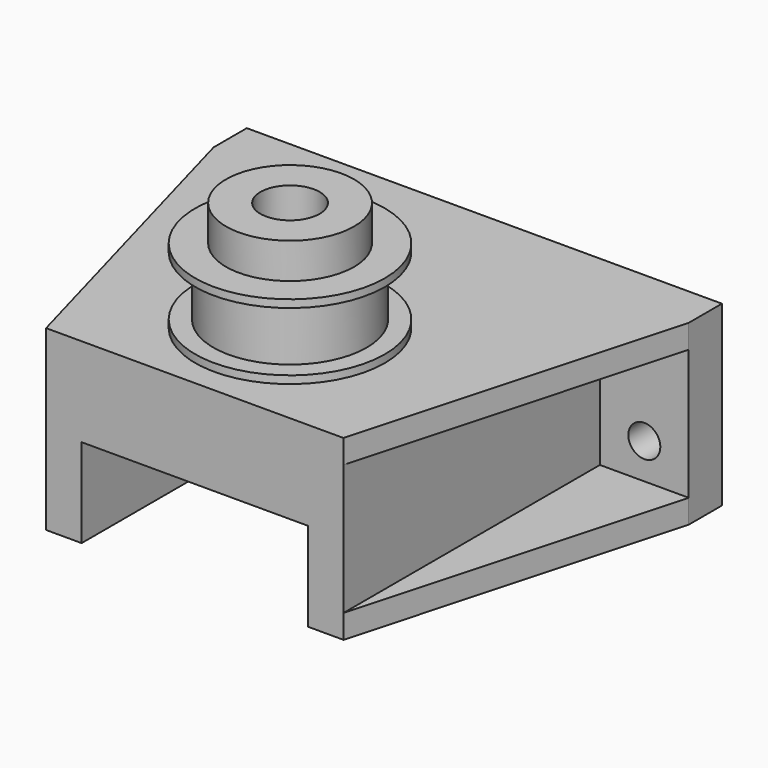
from build123d import *

# Parameters (mm, degrees)
F0_W              = 50.2
F0_H              = 61.1
F0_R              = 15.1
F1_DEPTH          = 15
F2_R              = 15
F2_R_2            = 5
F3_DEPTH          = 14
F5_DEPTH          = 15
F6_W              = 7
F6_H              = 30
F7_DEPTH          = 15
F8_R              = 2.7
F9_DEPTH          = 25
F11_DEPTH         = 4
F11_COPIES2_COUNT = 2
F12_R             = 16
F12_R_2           = 5
F13_DEPTH         = 1.3
F14_R             = 12.9361137745
F14_R_2           = 5
F15_DEPTH         = 10
F16_R             = 16
F16_R_2           = 5
F17_DEPTH         = 1.3
F18_R             = 10.8
F18_R_2           = 5
F19_DEPTH         = 6


# Not quite as in the source:
# - a pattern or mirror of a feature is missing from the dataset's text; its kind, count and spacing are read off the source's solid


with BuildPart() as f1:
    # F0 (on Top) → F1 (new body)
    with BuildSketch(Plane.XY):
        with Locations((0, 10.45)):
            Rectangle(F0_W, F0_H)
        Circle(F0_R, mode=Mode.SUBTRACT)
    extrude(amount=F1_DEPTH)

    # F4 (on face) → F5 (join)
    with BuildSketch(Plane(origin=(0, 0, 0), x_dir=(1, 0, 0), z_dir=(0, 0, -1))):
        Polygon((-25.1, 20.1), (-25.1, -41), (25.1, -41), (25.1, 20.1), (19.1, 20.1), (19.1, -20.1), (-19.1, -20.1), (-19.1, 20.1), align=None)
    extrude(amount=F5_DEPTH)

    # F6 (on face) → F7 (join)
    with BuildSketch(Plane(origin=(-25.1, 0, 0), x_dir=(0, -1, 0), z_dir=(-1, 0, 0))):
        with Locations((-37.5, 0)):
            Rectangle(F6_W, F6_H)
    f7 = extrude(amount=F7_DEPTH)

    # F7_copies: F7 across plane
    add(f7.mirror(Plane(origin=(0, 0, 0), x_dir=(0, 0, 1), z_dir=(1, 0, 0))))

    # F8 (on face) → F9 (cut)
    with BuildSketch(Plane.XZ.offset(-34)):
        with Locations((-32.6, -5)):
            Circle(F8_R)
    f9 = extrude(amount=-F9_DEPTH, mode=Mode.SUBTRACT)

    # F9_copies: F9 across plane
    add(f9.mirror(Plane(origin=(0, 0, 0), x_dir=(0, 0, 1), z_dir=(1, 0, 0))), mode=Mode.SUBTRACT)

    # F10 (on face) → F11 (join)
    with BuildSketch(Plane(origin=(0, 0, -15), x_dir=(1, 0, 0), z_dir=(0, 0, -1))):
        Polygon((-25.1, -34), (-25.1, 20.1), (-40.1, -34), align=None)
    f11 = extrude(amount=-F11_DEPTH)

    # F11_copies: F11 across plane
    add(f11.mirror(Plane.XY))

    # F11_copies1: F11 across plane
    add(f11.mirror(Plane(origin=(0, 0, 0), x_dir=(0, 0, 1), z_dir=(1, 0, 0))))

    # F11_copies2: F11 ×2 about axis
    f11_copies2_axis = Axis((0, 0, 0), (0, 1, 0))
    for i in range(1, F11_COPIES2_COUNT):
        add(f11.rotate(f11_copies2_axis, i * 360 / F11_COPIES2_COUNT))


with BuildPart() as f3:
    # F2 (on face) → F3 (new body)
    with BuildSketch(Plane.XY.offset(15)):
        Circle(F2_R)
        Circle(F2_R_2, mode=Mode.SUBTRACT)
    extrude(amount=-F3_DEPTH)


with BuildPart() as f13:
    # F12 (on face) → F13 (new body)
    with BuildSketch(Plane.XY.offset(15)):
        Circle(F12_R)
        Circle(F12_R_2, mode=Mode.SUBTRACT)
    extrude(amount=F13_DEPTH)

    # F14 (on face) → F15 (join)
    with BuildSketch(Plane.XY.offset(16.3)):
        Circle(F14_R)
        Circle(F14_R_2, mode=Mode.SUBTRACT)
    extrude(amount=F15_DEPTH)

    # F16 (on face) → F17 (join)
    with BuildSketch(Plane.XY.offset(26.3)):
        Circle(F16_R)
        Circle(F16_R_2, mode=Mode.SUBTRACT)
    extrude(amount=F17_DEPTH)

    # F18 (on face) → F19 (join)
    with BuildSketch(Plane.XY.offset(27.6)):
        Circle(F18_R)
        Circle(F18_R_2, mode=Mode.SUBTRACT)
    extrude(amount=F19_DEPTH)


solid = Compound([f1.part, f3.part, f13.part])
